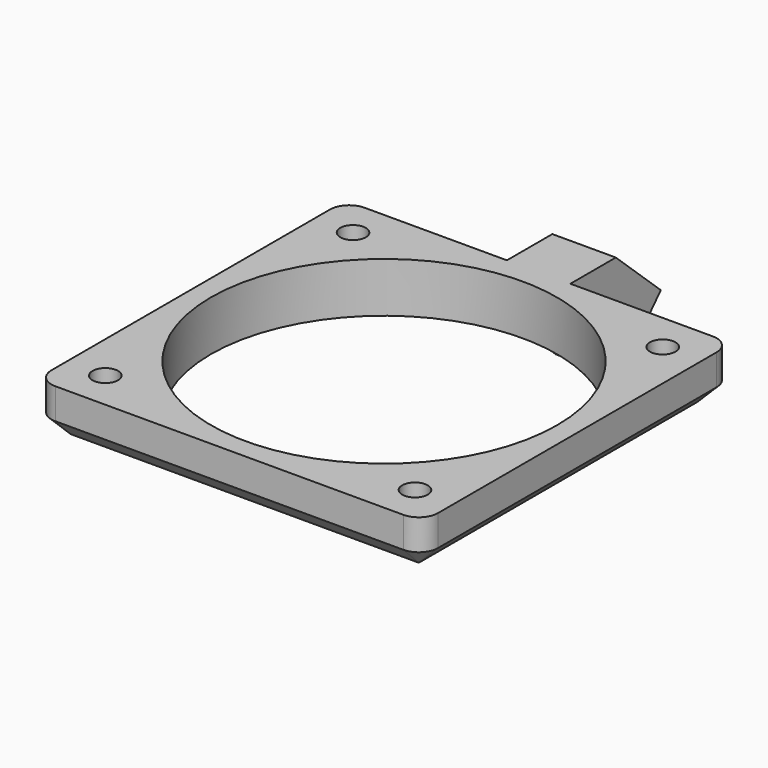
from build123d import *

# Parameters (mm, degrees)
F0_W     = 40.2
F0_H     = 40.2
F0_R     = 1.325
F0_R_2   = 18
F1_DEPTH = 5.2
F2_R     = 2
F6_DEPTH = 3.3
F7_SIZE  = 1.99999


# Not quite as in the source:
# - a fillet or chamfer is up to 0.001 mm smaller than in the source, because OpenCascade refuses the exact size


with BuildPart() as f1:
    # F0 (on Top) → F1 (new body)
    with BuildSketch(Plane.XY):
        Rectangle(F0_W, F0_H)
        with Locations((-16.1, -16.1)):
            Circle(F0_R, mode=Mode.SUBTRACT)
        with Locations((16.1, -16.1)):
            Circle(F0_R, mode=Mode.SUBTRACT)
        with Locations((-16.1, 16.1)):
            Circle(F0_R, mode=Mode.SUBTRACT)
        Circle(F0_R_2, mode=Mode.SUBTRACT)
        with Locations((16.1, 16.1)):
            Circle(F0_R, mode=Mode.SUBTRACT)
    extrude(amount=F1_DEPTH)

    # F2
    f2_edges = [f1.edges().sort_by_distance(p)[0] for p in [
        (-20.1, 20.1, 2.6),
        (20.1, 20.1, 2.6),
        (20.1, -20.1, 2.6),
        (-20.1, -20.1, 2.6),
    ]]
    fillet(f2_edges, radius=F2_R)

    # F5 (on line) → F6 (join, symmetric)
    with BuildSketch(Plane.YZ):
        Polygon((20.1, 5.2), (20.1, 0), (26.4531082501, -5.9914017233), (31.8527851563, -0.1601095172), (28.929274422, 2.5199452414), (26.0057636878, 5.2), align=None)
        with BuildLine():
            ThreePointArc((26.7126609223, -1.5342851533), (23.8396290954, -2.1382583334), (26.2262827859, -0.4285859547))
            ThreePointArc((26.2262827859, -0.4285859547), (26.5856927492, -0.9303119732), (26.7126609223, -1.5342851533))
        make_face(mode=Mode.SUBTRACT)
    extrude(amount=F6_DEPTH, both=True)

    # F7 (size 2 in the source; OpenCascade refuses exactly that, so slightly less here)
    f7_edges = [f1.edges().sort_by_distance(p)[0] for p in [
        (0, -20.1, 0),
    ]]
    chamfer(f7_edges, length=F7_SIZE)


solid = f1.part
